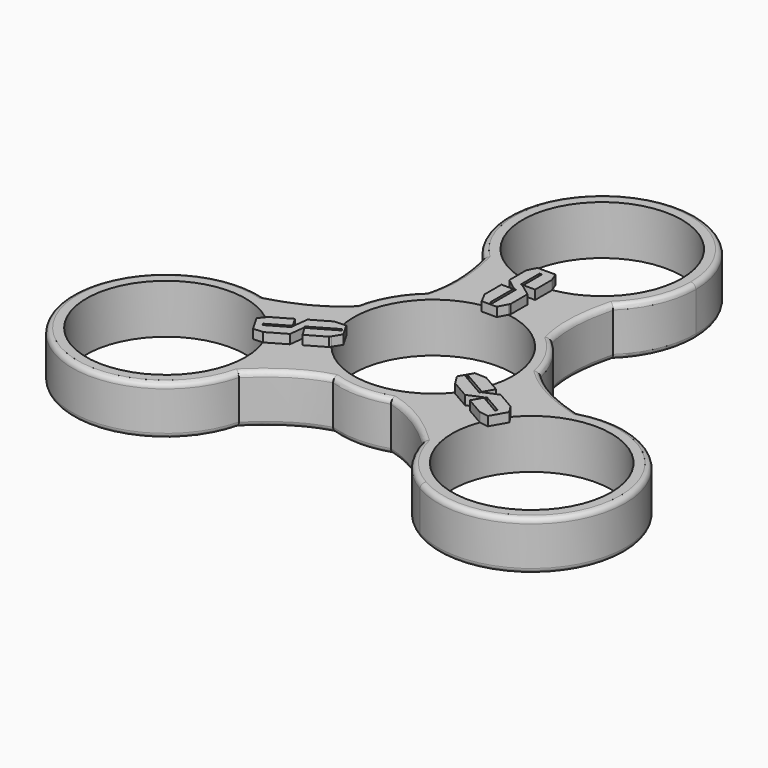
from build123d import *

# Parameters (mm, degrees)
F0_R     = 11.3
F1_DEPTH = 7
F2_COUNT = 3
F4_R     = 0.7242640687
F6_DEPTH = 1.3


# Not quite as in the source:
# - a feature names something its author has since deleted; it is built from what else it names


with BuildPart() as f1:
    # F0 (on Top) → F1 (new body)
    with BuildSketch(Plane.XY):
        with BuildLine():
            ThreePointArc((12.9868103729, -2.8692780169), (13.2214707571, -1.4431600813), (13.3, 0))
            ThreePointArc((13.3, 0), (12.1495384195, 5.4109810749), (8.8971855349, 9.885853001))
            add(Edge.make_bspline(
                [(8.8971855349, 9.885853001), (9.9206985939, 5.7179684341), (12.150645437, 1.6182620615), (12.9868103729, -2.8692780169)],
                knots=[0.5652103967, 0.5652103967, 0.5652103967, 0.5652103967, 0.9277941897, 0.9277941897, 0.9277941897, 0.9277941897], degree=3))
        make_face()
        with BuildLine():
            ThreePointArc((-9.2247815261, 20.4191129056), (2.414e-07, 16.7000001997), (9.2247820089, 20.4191129056))
            ThreePointArc((9.2247820089, 20.4191129056), (12.2388645169, 24.7942148366), (13.3000002414, 30.0000001997))
            ThreePointArc((13.3000002414, 30.0000001997), (-5.2057851216, 42.2388644752), (-9.2247815261, 20.4191129056))
        make_face()
        with Locations((2.414e-07, 30.0000001997)):
            Circle(F0_R, mode=Mode.SUBTRACT)
        with BuildLine():
            add(Edge.make_bspline(
                [(8.8971855349, 9.885853001), (9.9206985939, 5.7179684341), (12.150645437, 1.6182620615), (12.9868103729, -2.8692780169)],
                knots=[0.5652103967, 0.5652103967, 0.5652103967, 0.5652103967, 0.9277941897, 0.9277941897, 0.9277941897, 0.9277941897], degree=3))
            ThreePointArc((8.8971855349, 9.885853001), (4.169e-07, 13.3), (-8.8971849151, 9.8858535588))
            add(Edge.make_bspline(
                [(-8.8971849151, 9.8858535588), (-9.9206980023, 5.7179684329), (-12.1506453096, 1.6182615397), (-12.986810111, -2.8692792023)],
                knots=[0.5652103806, 0.5652103806, 0.5652103806, 0.5652103806, 0.9277942216, 0.9277942216, 0.9277942216, 0.9277942216], degree=3))
            ThreePointArc((-12.986810111, -2.8692792023), (6.07e-07, -13.3), (12.9868103729, -2.8692780169))
        make_face()
        Circle(F0_R, mode=Mode.SUBTRACT)
        with BuildLine():
            add(Edge.make_bspline(
                [(-8.8971849151, 9.8858535588), (-9.9206980023, 5.7179684329), (-12.1506453096, 1.6182615397), (-12.986810111, -2.8692792023)],
                knots=[0.5652103806, 0.5652103806, 0.5652103806, 0.5652103806, 0.9277942216, 0.9277942216, 0.9277942216, 0.9277942216], degree=3))
            ThreePointArc((-8.8971849151, 9.8858535588), (-12.6649383147, 4.0607065254), (-12.986810111, -2.8692792023))
        make_face()
        with BuildLine():
            ThreePointArc((-8.8971849151, 9.8858535588), (4.169e-07, 13.3), (8.8971855349, 9.885853001))
            add(Edge.make_bspline(
                [(9.2247820089, 20.4191129056), (8.5325194997, 17.6451609959), (8.0485337154, 14.0979107896), (8.7085584132, 10.6539683295), (8.8971855349, 9.885853001)],
                knots=[0.2665062134, 0.2665062134, 0.2665062134, 0.2665062134, 0.4983884479, 0.5652103967, 0.5652103967, 0.5652103967, 0.5652103967], degree=3))
            ThreePointArc((9.2247820089, 20.4191129056), (2.414e-07, 16.7000001997), (-9.2247815261, 20.4191129056))
            add(Edge.make_bspline(
                [(-9.2247815261, 20.4191129056), (-8.5325190169, 17.6451609959), (-8.0485332588, 14.0979109817), (-8.7085578589, 10.6539687025), (-8.8971849151, 9.8858535588)],
                knots=[0.2665062134, 0.2665062134, 0.2665062134, 0.2665062134, 0.4983884479, 0.5652103806, 0.5652103806, 0.5652103806, 0.5652103806], degree=3))
        make_face()
    extrude(amount=F1_DEPTH)


with BuildPart() as f2_1:
    # F2: instance of F1
    add(f1.part.rotate(Axis((0, 0, 0), (0, 0, -1)), 1 * 360 / F2_COUNT))


with BuildPart() as f2_2:
    # F2: instance of F1
    add(f1.part.rotate(Axis((0, 0, 0), (0, 0, -1)), 2 * 360 / F2_COUNT))


with BuildPart() as f1_1:
    add(f1.part)

    # F3: union F2_1, F2_2
    add(f2_1.part)
    add(f2_2.part)

    # F4
    f4_edges = [f1_1.edges().sort_by_distance(p)[0] for p in [
        (8.384284, 15.167432, 7),
        (11.518138, 6.65, 7),
        (8.943239, -14.844718, 7),
        (-17.327523, -0.322713, 7),
        (0, -13.3, 7),
        (0, -13.3, 0),
        (8.943239, -14.844718, 0),
        (11.518138, 6.65, 0),
        (8.384284, 15.167432, 0),
        (-17.327523, -0.322713, 0),
        (-37.4989, -21.65, 0),
        (-8.94324, -14.844718, 0),
        (-8.94324, -14.844718, 7),
        (-8.384283, 15.167432, 7),
        (-11.518138, 6.65, 7),
        (-37.4989, -21.65, 7),
        (37.4989, -21.65, 7),
        (17.327523, -0.322714, 7),
        (0, 43.3, 7),
        (-11.518138, 6.65, 0),
        (-8.384283, 15.167432, 0),
        (0, 43.3, 0),
        (17.327523, -0.322714, 0),
        (37.4989, -21.65, 0),
    ]]
    fillet(f4_edges, radius=F4_R)

    # F5 (on face) → F6 (join)
    with BuildSketch(Plane.XY.offset(7)):
        with BuildLine():
            Line((-0.1659937261, 11.2987807343), (-0.1659937261, 14.4068322358))
            Line((-0.1659937261, 14.4068322358), (-1.84583386, 14.4068322358))
            Line((-1.84583386, 14.4068322358), (-1.84583386, 11.4068322358))
            Line((-1.84583386, 11.4068322358), (-1.719393845, 11.1684235596))
            ThreePointArc((-1.719393845, 11.1684235596), (-0.9449443484, 11.2604209592), (-0.1659937261, 11.2987807343))
        make_face()
        with BuildLine():
            Line((1.820578386, 18.8074208079), (1.8056624332, 18.845199258))
            ThreePointArc((1.8056624332, 18.845199258), (0.9758422351, 18.7422147868), (0.1406785026, 18.7008759138))
            Line((0.1406785026, 18.7008759138), (0.1406785026, 15.831067088))
            Line((0.1406785026, 15.831067088), (-0.0293214974, 15.831067088))
            Line((-0.0293214974, 15.831067088), (-0.0293214974, 15.8074208079))
            Line((-0.0293214974, 15.8074208079), (1.820578386, 15.8074208079))
            Line((1.820578386, 15.8074208079), (1.820578386, 18.8074208079))
        make_face()
        with BuildLine():
            Line((-1.82517674, 18.8483756998), (-1.84583386, 18.8074208079))
            Line((-1.84583386, 18.8074208079), (-1.84583386, 15.8074208079))
            Line((-1.84583386, 15.8074208079), (-0.0550890274, 14.4516194639))
            Line((-0.0550890274, 14.4516194639), (0.1741257729, 14.4516194639))
            Line((0.1741257729, 14.4516194639), (0.1741257729, 11.298658337))
            ThreePointArc((0.1741257729, 11.298658337), (0.9527859808, 11.2597601606), (1.7269107753, 11.1672637282))
            Line((1.7269107753, 11.1672637282), (1.8539659067, 11.4068322358))
            Line((1.8539659067, 11.4068322358), (1.8539659067, 14.4068322358))
            Line((1.8539659067, 14.4068322358), (-0.0293214974, 15.8074208079))
            Line((-0.0293214974, 15.8074208079), (-0.0293214974, 15.831067088))
            Line((-0.0293214974, 15.831067088), (-0.1993214974, 15.831067088))
            Line((-0.1993214974, 15.831067088), (-0.1993214974, 18.7017582637))
            ThreePointArc((-0.1993214974, 18.7017582637), (-1.0149002144, 18.7456687195), (-1.82517674, 18.8483756998))
        make_face()
        with BuildLine():
            Line((-1.2262361591, 20.0358377815), (-1.82517674, 18.8483756998))
            ThreePointArc((-1.82517674, 18.8483756998), (-1.0149002144, 18.7456687195), (-0.1993214974, 18.7017582637))
            Line((-0.1993214974, 18.7017582637), (-0.1993214974, 19.1218581525))
            Line((-0.1993214974, 19.1218581525), (-0.0293214974, 19.1218581525))
            Line((-0.0293214974, 19.1218581525), (0.1406785026, 19.1218581525))
            Line((0.1406785026, 19.1218581525), (0.1406785026, 18.7008759138))
            ThreePointArc((0.1406785026, 18.7008759138), (0.9758422351, 18.7422147868), (1.8056624332, 18.845199258))
            Line((1.8056624332, 18.845199258), (1.3315546791, 20.0459979178))
            Line((1.3315546791, 20.0459979178), (-1.2262361591, 20.0358377815))
        make_face()
        with BuildLine():
            ThreePointArc((1.7269107753, 11.1672637282), (0.9527859808, 11.2597601606), (0.1741257729, 11.298658337))
            Line((0.1741257729, 11.298658337), (0.1741257729, 10.2516194639))
            Line((0.1741257729, 10.2516194639), (-0.1659937261, 10.2516194639))
            Line((-0.1659937261, 10.2516194639), (-0.1659937261, 11.2987807343))
            ThreePointArc((-0.1659937261, 11.2987807343), (-0.9449443484, 11.2604209592), (-1.719393845, 11.1684235596))
            Line((-1.719393845, 11.1684235596), (-1.0632626945, 9.9312569946))
            Line((-1.0632626945, 9.9312569946), (1.0713947412, 9.9312569946))
            Line((1.0713947412, 9.9312569946), (1.7269107753, 11.1672637282))
        make_face()
        with BuildLine():
            ThreePointArc((-9.8719880349, -5.4985318257), (-10.22763133, -4.8047432166), (-10.534589467, -4.0880832626))
            Line((-10.534589467, -4.0880832626), (-10.8055894463, -4.0978345449))
            Line((-10.8055894463, -4.0978345449), (-13.4036656577, -5.5978345449))
            Line((-13.4036656577, -5.5978345449), (-13.6749672392, -7.9291035655))
            Line((-13.6749672392, -7.9291035655), (-14.5999171809, -6.3270432721))
            Line((-14.5999171809, -6.3270432721), (-17.1979933923, -7.8270432721))
            Line((-17.1979933923, -7.8270432721), (-17.2232525134, -7.8588500912))
            ThreePointArc((-17.2232525134, -7.8588500912), (-16.7191552461, -8.5260032277), (-16.2657728657, -9.2286067999))
            Line((-16.2657728657, -9.2286067999), (-13.7804455186, -7.793702387))
            Line((-13.7804455186, -7.793702387), (-13.6104455186, -8.0881510243))
            Line((-13.6104455186, -8.0881510243), (-16.0965370031, -9.5234966121))
            ThreePointArc((-16.0965370031, -9.5234966121), (-15.7267752149, -10.2517637277), (-15.4105838061, -11.0048372731))
            Line((-15.4105838061, -11.0048372731), (-15.3647872693, -11.0022494179))
            Line((-15.3647872693, -11.0022494179), (-12.7667110579, -9.5022494179))
            Line((-12.7667110579, -9.5022494179), (-12.4879250679, -7.2735182292))
            Line((-12.4879250679, -7.2735182292), (-12.602532468, -7.0750123892))
            Line((-12.602532468, -7.0750123892), (-9.8719880349, -5.4985318257))
        make_face()
        with BuildLine():
            ThreePointArc((-8.8124416003, -7.0732505287), (-9.2793384338, -6.4485562905), (-9.7020342847, -5.7931451509))
            Line((-9.7020342847, -5.7931451509), (-12.3936858412, -7.3471709016))
            Line((-12.3936858412, -7.3471709016), (-11.5537657743, -8.8019551319))
            Line((-11.5537657743, -8.8019551319), (-8.9556895629, -7.3019551319))
            Line((-8.9556895629, -7.3019551319), (-8.8124416003, -7.0732505287))
        make_face()
        with BuildLine():
            Line((-9.1364182195, -4.0377734339), (-10.534589467, -4.0880832626))
            ThreePointArc((-10.534589467, -4.0880832626), (-10.22763133, -4.8047432166), (-9.8719880349, -5.4985318257))
            Line((-9.8719880349, -5.4985318257), (-8.9652257721, -4.9750123892))
            Line((-8.9652257721, -4.9750123892), (-8.7951660226, -5.2695645157))
            Line((-8.7951660226, -5.2695645157), (-9.7020342847, -5.7931451509))
            ThreePointArc((-9.7020342847, -5.7931451509), (-9.2793384338, -6.4485562905), (-8.8124416003, -7.0732505287))
            Line((-8.8124416003, -7.0732505287), (-8.0690895016, -5.8864410016))
            Line((-8.0690895016, -5.8864410016), (-9.1364182195, -4.0377734339))
        make_face()
        with BuildLine():
            ThreePointArc((-16.2657728657, -9.2286067999), (-16.7191552461, -8.5260032277), (-17.2232525134, -7.8588500912))
            Line((-17.2232525134, -7.8588500912), (-18.0261207806, -8.8698387803))
            Line((-18.0261207806, -8.8698387803), (-16.7384264253, -11.0798705556))
            Line((-16.7384264253, -11.0798705556), (-15.4105838061, -11.0048372731))
            ThreePointArc((-15.4105838061, -11.0048372731), (-15.7267752149, -10.2517637277), (-16.0965370031, -9.5234966121))
            Line((-16.0965370031, -9.5234966121), (-16.460354179, -9.7335465565))
            Line((-16.460354179, -9.7335465565), (-16.630354179, -9.4390979192))
            Line((-16.630354179, -9.4390979192), (-16.2657728657, -9.2286067999))
        make_face()
        with BuildLine():
            Line((12.4284066952, -7.3766070747), (9.697862262, -5.8001265112))
            ThreePointArc((9.697862262, -5.8001265112), (9.2748453492, -6.455016944), (8.8076786917, -7.0791804655))
            Line((8.8076786917, -7.0791804655), (8.9516235396, -7.3089976909))
            Line((8.9516235396, -7.3089976909), (11.5496997509, -8.8089976909))
            Line((11.5496997509, -8.8089976909), (13.7042887366, -7.8783172423))
            Line((13.7042887366, -7.8783172423), (12.7793387949, -9.4803775358))
            Line((12.7793387949, -9.4803775358), (15.3774150063, -10.9803775358))
            Line((15.3774150063, -10.9803775358), (15.4175900802, -10.9863491668))
            ThreePointArc((15.4175900802, -10.9863491668), (15.743313011, -10.2162115591), (16.1250943631, -9.472269114))
            Line((16.1250943631, -9.472269114), (13.6397670159, -8.0373647011))
            Line((13.6397670159, -8.0373647011), (13.8097670159, -7.7429160638))
            Line((13.8097670159, -7.7429160638), (16.2958585005, -9.1782616516))
            ThreePointArc((16.2958585005, -9.1782616516), (16.7416754292, -8.4939049918), (17.2357605461, -7.8435384267))
            Line((17.2357605461, -7.8435384267), (17.2106211293, -7.80517139))
            Line((17.2106211293, -7.80517139), (14.6125449179, -6.30517139))
            Line((14.6125449179, -6.30517139), (12.5430140953, -7.1781012348))
            Line((12.5430140953, -7.1781012348), (12.4284066952, -7.3766070747))
        make_face()
        with BuildLine():
            Line((10.801523423, -4.104877104), (10.5318354453, -4.0951730309))
            ThreePointArc((10.5318354453, -4.0951730309), (10.2242827822, -4.8118646687), (9.8680280108, -5.5056355835))
            Line((9.8680280108, -5.5056355835), (12.5596795674, -7.0596613342))
            Line((12.5596795674, -7.0596613342), (13.3995996343, -5.604877104))
            Line((13.3995996343, -5.604877104), (10.801523423, -4.104877104))
        make_face()
        with BuildLine():
            Line((17.9646625844, -8.9559672259), (17.2357605461, -7.8435384267))
            ThreePointArc((17.2357605461, -7.8435384267), (16.7416754292, -8.4939049918), (16.2958585005, -9.1782616516))
            Line((16.2958585005, -9.1782616516), (16.6596756763, -9.388311596))
            Line((16.6596756763, -9.388311596), (16.4896756763, -9.6827602333))
            Line((16.4896756763, -9.6827602333), (16.1250943631, -9.472269114))
            ThreePointArc((16.1250943631, -9.472269114), (15.743313011, -10.2162115591), (15.4175900802, -10.9863491668))
            Line((15.4175900802, -10.9863491668), (16.6945661015, -11.1761591375))
            Line((16.6945661015, -11.1761591375), (17.9646625844, -8.9559672259))
        make_face()
        with BuildLine():
            ThreePointArc((9.8680280108, -5.5056355835), (10.2242827822, -4.8118646687), (10.5318354453, -4.0951730309))
            Line((10.5318354453, -4.0951730309), (9.1323521961, -4.044815993))
            Line((9.1323521961, -4.044815993), (8.0650234782, -5.8934835607))
            Line((8.0650234782, -5.8934835607), (8.8076786917, -7.0791804655))
            ThreePointArc((8.8076786917, -7.0791804655), (9.2748453492, -6.455016944), (9.697862262, -5.8001265112))
            Line((9.697862262, -5.8001265112), (8.7910999993, -5.2766070747))
            Line((8.7910999993, -5.2766070747), (8.9611597488, -4.9820549483))
            Line((8.9611597488, -4.9820549483), (9.8680280108, -5.5056355835))
        make_face()
    extrude(amount=F6_DEPTH)


solid = f1_1.part
